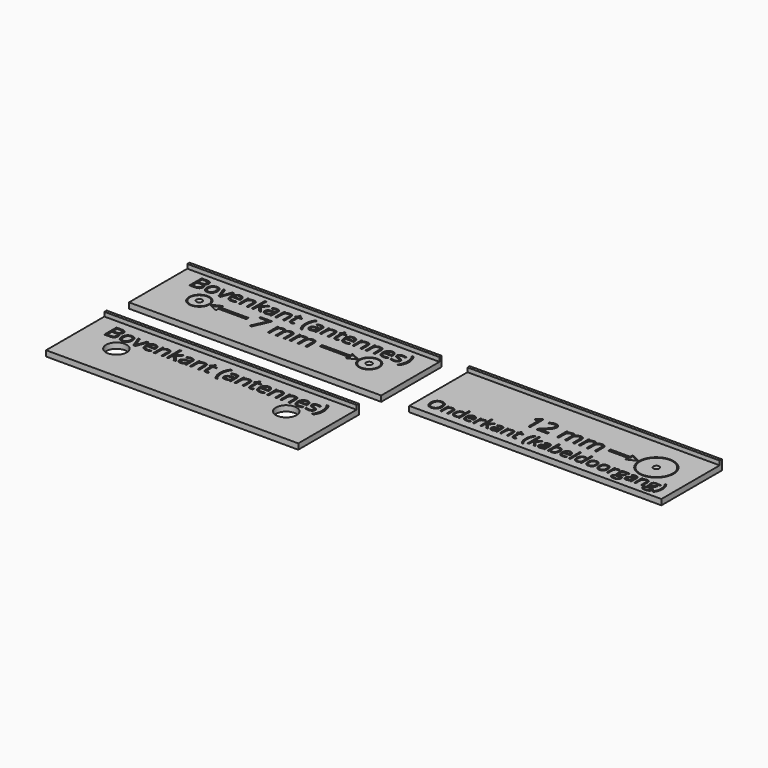
from build123d import *

# Parameters (mm, degrees)
F0_W                     = 90
F0_H                     = 27
F1_DEPTH                 = 2
F0_R                     = 3.7
F2_R                     = 1.05
F3_DEPTH                 = 25
DRAFT_F3_DRAFTED_ANGLE   = 14
DRAFT_F3_2_DRAFTED_ANGLE = 14
DRAFT_F3_3_DRAFTED_ANGLE = 14
F2_R_2                   = 3.675
F2_R_3                   = 3.325
F2_TEXT_SIZE             = 7.6458875785
F2_TEXT_SIZE_2           = 8.3333333333
F2_R_4                   = 6.175
F2_R_5                   = 5.825
F2_TEXT_SIZE_3           = 6.5109181412
F4_DEPTH                 = 0.4
F2_W                     = 90
F2_H                     = 1
F5_DEPTH                 = 1.5


# Not quite as in the source:
# - an extrude with a draft is written as a straight extrude whose walls are then drafted
# - Text() gives the source's letters only with a copy of the font that has no kerning and outlines rounded to 1/6400 em; it was checked with that copy


with BuildPart() as f1:
    # F0 (on Top) → F1 (new body)
    with BuildSketch(Plane.XY):
        Rectangle(F0_W, F0_H)
    extrude(amount=F1_DEPTH)


with BuildPart() as f1b:
    # F0 (on Top) → F1, piece 2 (new body)
    with BuildSketch(Plane.XY):
        with Locations((0, -37)):
            Rectangle(F0_W, F0_H)
        with Locations((-30.3, -37.5)):
            Circle(F0_R, mode=Mode.SUBTRACT)
        with Locations((30.3, -37.5)):
            Circle(F0_R, mode=Mode.SUBTRACT)
    extrude(amount=F1_DEPTH)


with BuildPart() as f1c:
    # F0 (on Top) → F1, piece 3 (new body)
    with BuildSketch(Plane.XY):
        with Locations((100, 0)):
            Rectangle(F0_W, F0_H)
    extrude(amount=F1_DEPTH)


with BuildPart() as f3_drafted:
    # F2 (on face) → F3 (new body)
    with BuildSketch(Plane.XY.offset(2)):
        with Locations((-30.3, -0.5)):
            Circle(F2_R)
    extrude(amount=-F3_DEPTH)

    # draft_F3_drafted
    draft_f3_drafted_walls = [f3_drafted.faces().sort_by_distance(p)[0] for p in [
        (-31.35, -0.5, -14.6666666667),
    ]]
    draft(draft_f3_drafted_walls, neutral_plane=Plane(origin=(0, 0, 2), x_dir=(1, 0, 0), z_dir=(0, 0, -1)), angle=DRAFT_F3_DRAFTED_ANGLE)


with BuildPart() as f1_1:
    add(f1.part)

    # join_F3_drafted: cut F3_drafted
    add(f3_drafted.part, mode=Mode.SUBTRACT)


with BuildPart() as f3_2_drafted:
    # F2 (on face) → F3, piece 2 (new body)
    with BuildSketch(Plane.XY.offset(2)):
        with Locations((30.3, -0.5)):
            Circle(F2_R)
    extrude(amount=-F3_DEPTH)

    # draft_F3_2_drafted
    draft_f3_2_drafted_walls = [f3_2_drafted.faces().sort_by_distance(p)[0] for p in [
        (29.25, -0.5, -14.6666666667),
    ]]
    draft(draft_f3_2_drafted_walls, neutral_plane=Plane(origin=(0, 0, 2), x_dir=(1, 0, 0), z_dir=(0, 0, -1)), angle=DRAFT_F3_2_DRAFTED_ANGLE)


with BuildPart() as f1_2:
    add(f1_1.part)

    # join_F3_2_drafted: cut F3_2_drafted
    add(f3_2_drafted.part, mode=Mode.SUBTRACT)


with BuildPart() as f3_3_drafted:
    # F2 (on face) → F3, piece 3 (new body)
    with BuildSketch(Plane.XY.offset(2)):
        with Locations((132, 0.5)):
            Circle(F2_R)
    extrude(amount=-F3_DEPTH)

    # draft_F3_3_drafted
    draft_f3_3_drafted_walls = [f3_3_drafted.faces().sort_by_distance(p)[0] for p in [
        (130.95, 0.5, -14.6666666667),
    ]]
    draft(draft_f3_3_drafted_walls, neutral_plane=Plane(origin=(0, 0, 2), x_dir=(1, 0, 0), z_dir=(0, 0, -1)), angle=DRAFT_F3_3_DRAFTED_ANGLE)


with BuildPart() as f1c_1:
    add(f1c.part)

    # join_F3_3_drafted: cut F3_3_drafted
    add(f3_3_drafted.part, mode=Mode.SUBTRACT)


with BuildPart() as f4_tool:
    # F2 (on face) → F4 (new body)
    with BuildSketch(Plane.XY.offset(2)):
        with Locations((-30.3, -0.5)):
            Circle(F2_R_2)
        with Locations((-30.3, -0.5)):
            Circle(F2_R_3, mode=Mode.SUBTRACT)
        with Locations((30.3, -0.5)):
            Circle(F2_R_2)
        with Locations((30.3, -0.5)):
            Circle(F2_R_3, mode=Mode.SUBTRACT)
        with Locations((-39, 4.9949609435)):
            Text('Bovenkant (antennes)', F2_TEXT_SIZE, font='Open Sans', text_align=(TextAlign.LEFT, TextAlign.BOTTOM))
        with Locations((-39, -33.0050390565)):
            Text('Bovenkant (antennes)', F2_TEXT_SIZE, font='Open Sans', text_align=(TextAlign.LEFT, TextAlign.BOTTOM))
        Polygon((-23.0985168517, 1.1320768035), (-26.5985168517, -0.5), (-23.0985168517, -2.1320768035), (-23.0985168517, -1), (-13.0985168517, -1), (-13.0985168517, 0), (-23.0985168517, 0), align=None)
        with Locations((-11.1484375, -3.5)):
            Text('7 mm', F2_TEXT_SIZE_2, font='Open Sans', text_align=(TextAlign.LEFT, TextAlign.BOTTOM))
        Polygon((23.0985168517, -2.1320768035), (26.5985168517, -0.5), (23.0985168517, 1.1320768035), (23.0985168517, 0), (13.0985168517, 0), (13.0985168517, -1), (23.0985168517, -1), align=None)
        Polygon((122.2453262806, -1.1320768035), (125.7453262806, 0.5), (122.2453262806, 2.1320768035), (122.2453262806, 1), (115.2453262806, 1), (115.2453262806, 0), (122.2453262806, 0), align=None)
        with Locations((132, 0.5)):
            Circle(F2_R_4)
        with Locations((132, 0.5)):
            Circle(F2_R_5, mode=Mode.SUBTRACT)
        with Locations((86.4694010417, -2.5)):
            Text('12 mm', F2_TEXT_SIZE_2, font='Open Sans', text_align=(TextAlign.LEFT, TextAlign.BOTTOM))
        with Locations((58, -10.5)):
            Text('Onderkant (kabeldoorgang)', F2_TEXT_SIZE_3, font='Open Sans', text_align=(TextAlign.LEFT, TextAlign.BOTTOM))
    extrude(amount=-F4_DEPTH)


with BuildPart() as f1_3:
    add(f1_2.part)

    # F4: cut by f4_tool
    add(f4_tool.part, mode=Mode.SUBTRACT)

    # F2 (on face) → F5 (join)
    with BuildSketch(Plane.XY.offset(2)):
        with Locations((0, 13)):
            Rectangle(F2_W, F2_H)
    extrude(amount=F5_DEPTH)


with BuildPart() as f1b_1:
    add(f1b.part)

    # F4: cut by f4_tool
    add(f4_tool.part, mode=Mode.SUBTRACT)

    # F2 (on face) → F5, piece 2 (join)
    with BuildSketch(Plane.XY.offset(2)):
        with Locations((0, -24)):
            Rectangle(F2_W, F2_H)
    extrude(amount=F5_DEPTH)


with BuildPart() as f1c_2:
    add(f1c_1.part)

    # F4: cut by f4_tool
    add(f4_tool.part, mode=Mode.SUBTRACT)

    # F2 (on face) → F5, piece 3 (join)
    with BuildSketch(Plane.XY.offset(2)):
        with Locations((100, 13)):
            Rectangle(F2_W, F2_H)
    extrude(amount=F5_DEPTH)


solid = Compound([f1_3.part, f1b_1.part, f1c_2.part])
